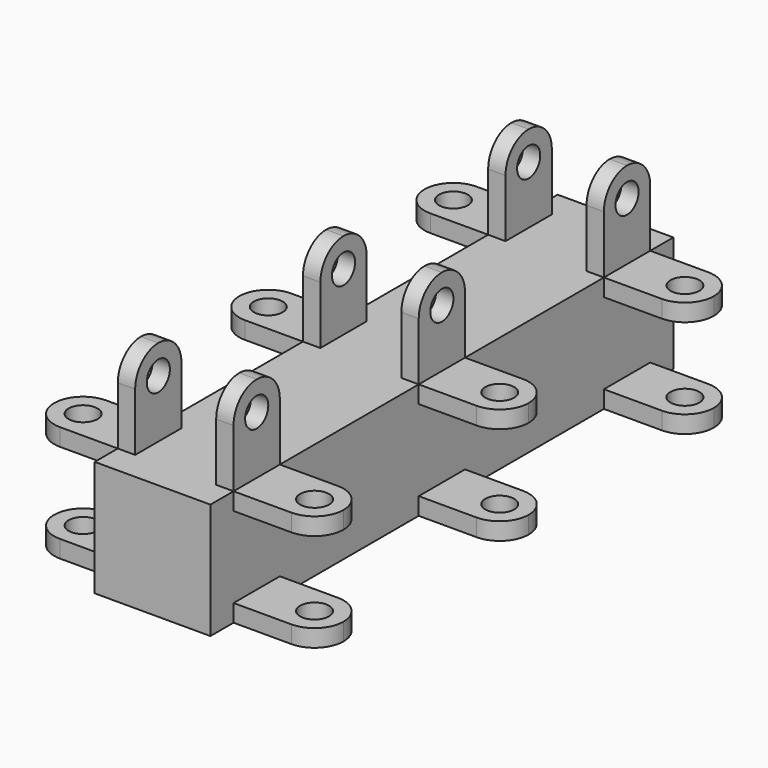
from build123d import *

# Parameters (mm, degrees)
F0_W          = 20
F0_H          = 20
F1_DEPTH      = 50
F2_W          = 10
F2_H          = 3
F3_DEPTH      = 25
F3_DEPTH_BACK = 25
F4_R          = 4.99999
F5_R          = 2.5
F6_DEPTH      = 10
F7_R          = 4.99999
F8_W          = 3
F8_H          = 10
F9_DEPTH      = 25
F10_R         = 4.99999
F12_DEPTH     = 25
F13_R         = 4.99999
F11_R         = 2.5
F14_DEPTH     = 10


# Not quite as in the source:
# - a fillet or chamfer is up to 0.001 mm smaller than in the source, because OpenCascade refuses the exact size
# - a feature names something its author has since deleted; it is built from what else it names


with BuildPart() as f1:
    # F0 (on Front) → F1 (new body, symmetric)
    with BuildSketch(Plane.XZ):
        Rectangle(F0_W, F0_H)
    extrude(amount=F1_DEPTH, both=True)

    # F2 (on Right) → F3 (join, two sides)
    with BuildSketch(Plane.YZ) as f3_sk:
        with Locations((-40, 8.5)):
            Rectangle(F2_W, F2_H)
        with Locations((-40, -8.5)):
            Rectangle(F2_W, F2_H)
        with Locations((40, -8.5)):
            Rectangle(F2_W, F2_H)
        with Locations((40, 8.5)):
            Rectangle(F2_W, F2_H)
        with Locations((0, 8.5)):
            Rectangle(F2_W, F2_H)
        with Locations((0, -8.5)):
            Rectangle(F2_W, F2_H)
    extrude(amount=F3_DEPTH)
    extrude(f3_sk.sketch, amount=-F3_DEPTH_BACK)

    # F4 (radius 5 in the source; OpenCascade refuses exactly that, so slightly less here)
    f4_edges = [f1.edges().sort_by_distance(p)[0] for p in [
        (25, -45, 8.5),
        (25, -35, 8.5),
        (25, -45, -8.5),
        (25, -35, -8.5),
        (25, -5, 8.5),
        (25, 5, 8.5),
        (25, -5, -8.5),
        (25, 5, -8.5),
        (25, 35, 8.5),
        (25, 45, 8.5),
        (25, 35, -8.5),
        (25, 45, -8.5),
    ]]
    fillet(f4_edges, radius=F4_R)

    # F5 (on Top) → F6 (cut, symmetric)
    with BuildSketch(Plane.XY):
        with Locations((20, -40)):
            Circle(F5_R)
        with Locations((20, 40)):
            Circle(F5_R)
        with Locations((20, 0)):
            Circle(F5_R)
        with Locations((-20, -40)):
            Circle(F5_R)
        with Locations((-20, 0)):
            Circle(F5_R)
        with Locations((-20, 40)):
            Circle(F5_R)
    extrude(amount=F6_DEPTH, both=True, mode=Mode.SUBTRACT)

    # F7 (radius 5 in the source; OpenCascade refuses exactly that, so slightly less here)
    f7_edges = [f1.edges().sort_by_distance(p)[0] for p in [
        (-25, -45, -8.5),
        (-25, -35, -8.5),
        (-25, -45, 8.5),
        (-25, -35, 8.5),
        (-25, -5, -8.5),
        (-25, 5, -8.5),
        (-25, -5, 8.5),
        (-25, 5, 8.5),
        (-25, 35, -8.5),
        (-25, 45, -8.5),
        (-25, 35, 8.5),
        (-25, 45, 8.5),
    ]]
    fillet(f7_edges, radius=F7_R)

    # F8 (on Top) → F9 (join)
    with BuildSketch(Plane.XY):
        with Locations((8.5, 0)):
            Rectangle(F8_W, F8_H)
        with Locations((-8.5, 0)):
            Rectangle(F8_W, F8_H)
        with Locations((8.5, 40)):
            Rectangle(F8_W, F8_H)
        with Locations((-8.5, 40)):
            Rectangle(F8_W, F8_H)
        with Locations((-8.5, -40)):
            Rectangle(F8_W, F8_H)
        with Locations((8.5, -40)):
            Rectangle(F8_W, F8_H)
    extrude(amount=F9_DEPTH)

    # F10 (radius 5 in the source; OpenCascade refuses exactly that, so slightly less here)
    f10_edges = [f1.edges().sort_by_distance(p)[0] for p in [
        (8.5, -5, 25),
        (8.5, 5, 25),
        (-8.5, -5, 25),
        (-8.5, 5, 25),
    ]]
    fillet(f10_edges, radius=F10_R)

    # F8 (on Top) → F12 (join)
    with BuildSketch(Plane.XY):
        with Locations((8.5, 0)):
            Rectangle(F8_W, F8_H)
        with Locations((-8.5, 0)):
            Rectangle(F8_W, F8_H)
        with Locations((8.5, 40)):
            Rectangle(F8_W, F8_H)
        with Locations((-8.5, 40)):
            Rectangle(F8_W, F8_H)
        with Locations((-8.5, -40)):
            Rectangle(F8_W, F8_H)
        with Locations((8.5, -40)):
            Rectangle(F8_W, F8_H)
    extrude(amount=F12_DEPTH)

    # F13 (radius 5 in the source; OpenCascade refuses exactly that, so slightly less here)
    f13_edges = [f1.edges().sort_by_distance(p)[0] for p in [
        (8.5, 45, 25),
        (-8.5, 45, 25),
        (-8.5, 35, 25),
        (8.5, 35, 25),
        (8.5, 5, 25),
        (8.5, -5, 25),
        (-8.5, 5, 25),
        (-8.5, -5, 25),
        (8.5, -35, 25),
        (8.5, -45, 25),
        (-8.5, -35, 25),
        (-8.5, -45, 25),
    ]]
    fillet(f13_edges, radius=F13_R)

    # F11 (on Right) → F14 (cut, symmetric)
    with BuildSketch(Plane.YZ):
        with Locations((-40, 20)):
            Circle(F11_R)
        with Locations((40, 20)):
            Circle(F11_R)
        with Locations((0, 20)):
            Circle(F11_R)
    extrude(amount=F14_DEPTH, both=True, mode=Mode.SUBTRACT)


solid = f1.part
